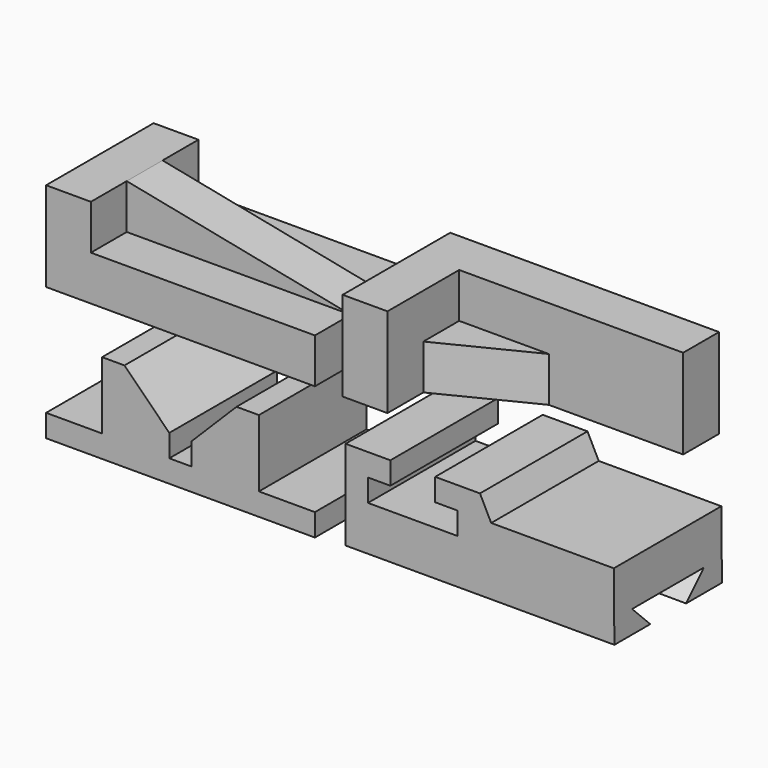
from build123d import *

# Parameters (mm, degrees)
F1_DEPTH  = 76.2
F2_DEPTH  = 76.2
F3_W      = 129.5150956453
F3_H      = 25.4
F4_DEPTH  = 25.4
F5_DEPTH  = 25.4
F6_W      = 127
F6_H      = 50.8
F7_DEPTH  = 25.4
F6_W_2    = 25.4
F8_DEPTH  = 76.2
F9_W      = 50.8
F9_H      = 25.4
F10_DEPTH = 25.4
F12_DEPTH = 25.4
F15_DEPTH = 76.2
F16_DEPTH = 76.2
F18_DEPTH = 152.4


with BuildPart() as f1:
    # F0 (on Front) → F1 (new body)
    with BuildSketch(Plane.XZ):
        Polygon((0, 50.8), (0, 0), (152.4, 0), (152.4, 25.4), (25.4, 25.4), (25.4, 50.8), align=None)
    extrude(amount=F1_DEPTH)


with BuildPart() as f2:
    # F0 (on Front) → F2 (new body)
    with BuildSketch(Plane.XZ):
        Polygon((25.4, 25.4), (152.4, 25.4), (25.4, 50.8), align=None)
    extrude(amount=F2_DEPTH)

    # F3 (on face) → F4 (cut)
    with BuildSketch(Plane(origin=(10.7461538462, 0, 53.7307692308), x_dir=(0.9805806757, 0, -0.1961161351), z_dir=(0.1961161351, 0, 0.9805806757))):
        with Locations((79.7015973202, -63.5)):
            Rectangle(F3_W, F3_H)
    extrude(amount=-F4_DEPTH, mode=Mode.SUBTRACT)

    # F3 (on face) → F5 (cut)
    with BuildSketch(Plane(origin=(10.7461538462, 0, 53.7307692308), x_dir=(0.9805806757, 0, -0.1961161351), z_dir=(0.1961161351, 0, 0.9805806757))):
        with Locations((79.7015973202, -12.7)):
            Rectangle(F3_W, F3_H)
    extrude(amount=-F5_DEPTH, mode=Mode.SUBTRACT)


with BuildPart() as f7:
    # F6 (on Front) → F7 (new body)
    with BuildSketch(Plane.XZ):
        with Locations((257.0362193159, 25.4)):
            Rectangle(F6_W, F6_H)
    extrude(amount=F7_DEPTH)

    # F6 (on Front) → F8 (join)
    with BuildSketch(Plane.XZ):
        with Locations((180.8362193159, 25.4)):
            Rectangle(F6_W_2, F6_H)
    extrude(amount=F8_DEPTH)

    # F9 (on face) → F10 (join)
    with BuildSketch(Plane.XZ.offset(25.4)):
        with Locations((218.9362193159, 12.7)):
            Rectangle(F9_W, F9_H)
    extrude(amount=F10_DEPTH)

    # F11 (on face) → F12 (cut)
    with BuildSketch(Plane.XY.offset(25.4)):
        Polygon((244.3362193159, -25.4), (193.5362193159, -50.8), (244.3362193159, -50.8), align=None)
    extrude(amount=-F12_DEPTH, mode=Mode.SUBTRACT)


with BuildPart() as f15:
    # F13 (on Front) → F15 (new body)
    with BuildSketch(Plane.XZ):
        Polygon((0, -62.7732424857), (0, -75.4732424857), (152.4, -75.4732424857), (152.4, -62.7732424857), (120.65, -62.7732424857), (120.65, -24.6732424857), (107.95, -24.6732424857), (82.55, -50.0732424857), (82.55, -62.7732424857), (69.85, -62.7732424857), (69.85, -50.0732424857), (44.45, -24.6732424857), (31.75, -24.6732424857), (31.75, -62.7732424857), align=None)
    extrude(amount=F15_DEPTH)


with BuildPart() as f16:
    # F14 (on Front) → F16 (new body)
    with BuildSketch(Plane.XZ):
        Polygon((169.773291292, -23.0053452725), (169.773291292, -73.8053452725), (322.173291292, -73.8053452725), (321.8548595905, -35.7053452725), (252.323291292, -35.7053452725), (245.973291292, -23.0053452725), (220.573291292, -23.0053452725), (220.573291292, -35.7053452725), (233.273291292, -35.7053452725), (233.273291292, -48.4053452725), (182.473291292, -48.4053452725), (182.473291292, -35.7053452725), (195.173291292, -35.7053452725), (195.173291292, -23.0053452725), align=None)
    extrude(amount=F16_DEPTH)

    # F17 (on face) → F18 (cut)
    with BuildSketch(Plane(origin=(321.5339819162, 0, 2.6873126754), x_dir=(0, 1, 0), z_dir=(0.9999650755, 0, 0.0083574955))):
        Polygon((-63.5, -63.7953295072), (-50.8, -76.4953295072), (-25.4, -76.4953295072), (-12.7, -63.7953295072), align=None)
    extrude(amount=-F18_DEPTH, mode=Mode.SUBTRACT)


solid = Compound([f1.part, f2.part, f7.part, f15.part, f16.part])
